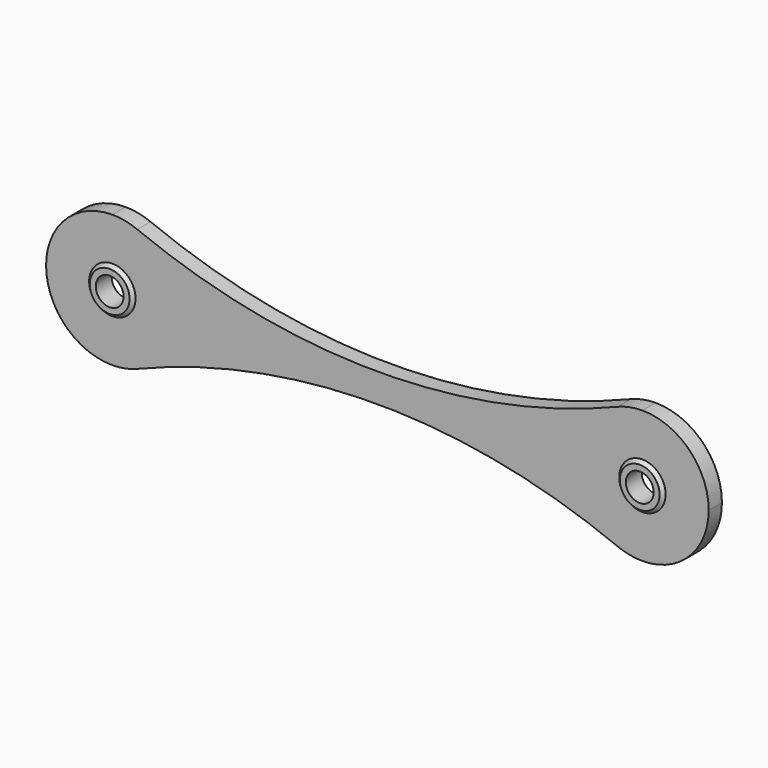
from build123d import *

# Parameters (mm, degrees)
F0_R     = 6
F1_DEPTH = 2.5
F2_DEPTH = 3
F2_TAPER = 45
F3_D     = 4.2
F4_R     = 9.99999


# Not quite as in the source:
# - a fillet or chamfer is up to 0.001 mm smaller than in the source, because OpenCascade refuses the exact size


with BuildPart() as f1:
    # F0 (on Front) → F1 (new body)
    with BuildSketch(Plane.XZ):
        with BuildLine():
            Line((-50, 16.2119245403), (-50, -10))
            Line((-50, -10), (50, -10))
            Line((50, -10), (50, 16.2119245403))
            ThreePointArc((50, 16.2119245403), (0, 2.1631295345), (-50, 16.2119245403))
        make_face()
        with Locations((-40, 0)):
            Circle(F0_R, mode=Mode.SUBTRACT)
        with Locations((40, 0)):
            Circle(F0_R, mode=Mode.SUBTRACT)
        with Locations((-40, 0)):
            Circle(F0_R)
        with Locations((40, 0)):
            Circle(F0_R)
    extrude(amount=F1_DEPTH)

    # F0 (on Front) → F2 (join)
    with BuildSketch(Plane.XZ):
        with Locations((40, 0)):
            Circle(F0_R)
        with Locations((-40, 0)):
            Circle(F0_R)
    extrude(amount=F2_DEPTH, taper=F2_TAPER)

    # F3 (through all)
    with Locations(Plane(origin=(0, 0, 0), x_dir=(1, 0, 0), z_dir=(0, 1, 0))):
        with Locations((40, 0), (-40, 0)):
            Hole(F3_D / 2)

    # F4 (radius 10 in the source; OpenCascade refuses exactly that, so slightly less here)
    f4_edges = [f1.edges().sort_by_distance(p)[0] for p in [
        (-50, -1.25, 16.211925),
        (50, -1.25, 16.211925),
        (50, -1.25, -10),
        (-50, -1.25, -10),
    ]]
    fillet(f4_edges, radius=F4_R)


with BuildPart() as f5_1:
    # F5: instance of F1
    add(f1.part.mirror(Plane.XY))


with BuildPart() as f1_1:
    add(f1.part)

    # F6: intersect F5_1
    add(f5_1.part, mode=Mode.INTERSECT)


solid = f1_1.part
